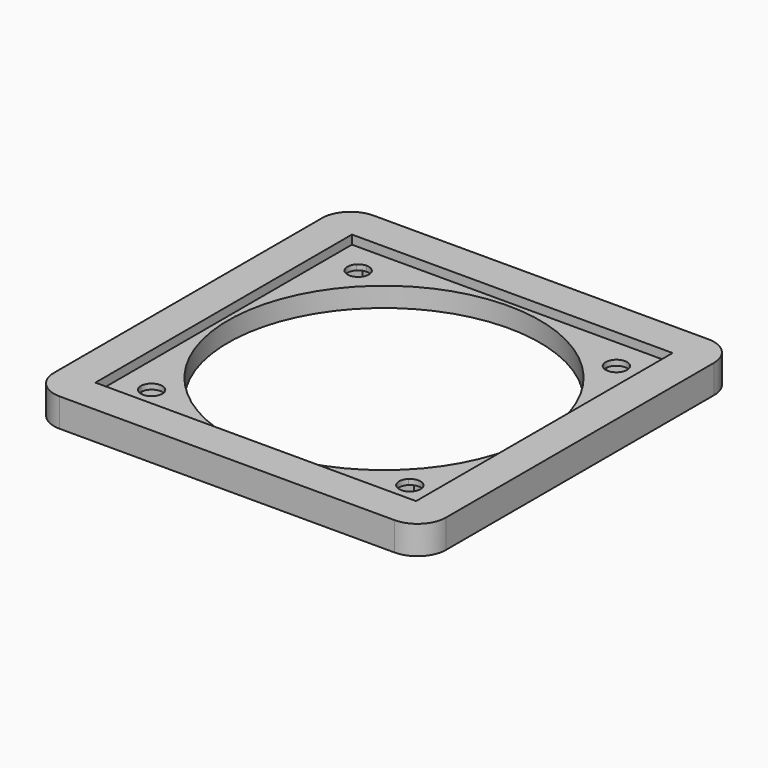
from build123d import *

# Parameters (mm, degrees)
F0_W             = 69.85
F0_H             = 69.85
F1_DEPTH         = 5.08
F2_R             = 5.08
F3_R             = 27.78125
F4_DEPTH         = 5.08
F5_W             = 57.15
F5_H             = 57.15
F6_DEPTH         = 1.5875
F8_DEPTH         = 3.4925
F8_COPIES_COUNT  = 4
F11_DEPTH        = 2.54
F11_COPIES_COUNT = 4


# Not quite as in the source:
# - a pattern or mirror of a feature is missing from the dataset's text; its kind, count and spacing are read off the source's solid


with BuildPart() as f1:
    # F0 (on Top) → F1 (new body)
    with BuildSketch(Plane.XY):
        Rectangle(F0_W, F0_H)
    extrude(amount=F1_DEPTH)

    # F2
    f2_edges = [f1.edges().sort_by_distance(p)[0] for p in [
        (-34.925, -34.925, 2.54),
        (34.925, -34.925, 2.54),
        (34.925, 34.925, 2.54),
        (-34.925, 34.925, 2.54),
    ]]
    fillet(f2_edges, radius=F2_R)

    # F3 (on face) → F4 (cut, through all)
    with BuildSketch(Plane.XY.offset(5.08)):
        Circle(F3_R)
    extrude(amount=-F4_DEPTH, mode=Mode.SUBTRACT)

    # F5 (on face) → F6 (cut)
    with BuildSketch(Plane.XY.offset(5.08)):
        Rectangle(F5_W, F5_H)
    extrude(amount=-F6_DEPTH, mode=Mode.SUBTRACT)

    # F7 (on face) → F8 (cut, through all)
    with BuildSketch(Plane.XY.offset(3.4925)):
        with BuildLine():
            Line((21.6602027868, 21.6602027868), (24.3542796231, 24.3542796231))
            ThreePointArc((24.3542796231, 24.3542796231), (21.6602027868, 24.3542796231), (21.6602027868, 21.6602027868))
        make_face()
        with BuildLine():
            ThreePointArc((24.9122412049, 23.0072412049), (24.7672317144, 23.7362531436), (24.3542796231, 24.3542796231))
            Line((24.3542796231, 24.3542796231), (21.6602027868, 21.6602027868))
            ThreePointArc((21.6602027868, 21.6602027868), (23.7362531436, 21.2472506955), (24.9122412049, 23.0072412049))
        make_face()
    f8 = extrude(amount=-F8_DEPTH, mode=Mode.SUBTRACT)

    # F8_copies: F8 ×4 about axis
    f8_copies_axis = Axis((0, 0, 0), (0, 0, 1))
    for i in range(1, F8_COPIES_COUNT):
        add(f8.rotate(f8_copies_axis, i * 360 / F8_COPIES_COUNT), mode=Mode.SUBTRACT)

    # F10 (on face) → F11 (cut)
    with BuildSketch(Plane(origin=(0, 0, 0), x_dir=(1, 0, 0), z_dir=(0, 0, -1))):
        Polygon((26.8172412049, 23.0072412049), (24.9122412049, 26.3067979934), (21.1022412049, 26.3067979934), (19.1972412049, 23.0072412049), (21.1022412049, 19.7076844165), (24.9122412049, 19.7076844165), align=None)
    f11 = extrude(amount=-F11_DEPTH, mode=Mode.SUBTRACT)

    # F11_copies: F11 ×4 about axis
    f11_copies_axis = Axis((0, 0, 0), (0, 0, 1))
    for i in range(1, F11_COPIES_COUNT):
        add(f11.rotate(f11_copies_axis, i * 360 / F11_COPIES_COUNT), mode=Mode.SUBTRACT)


solid = f1.part
